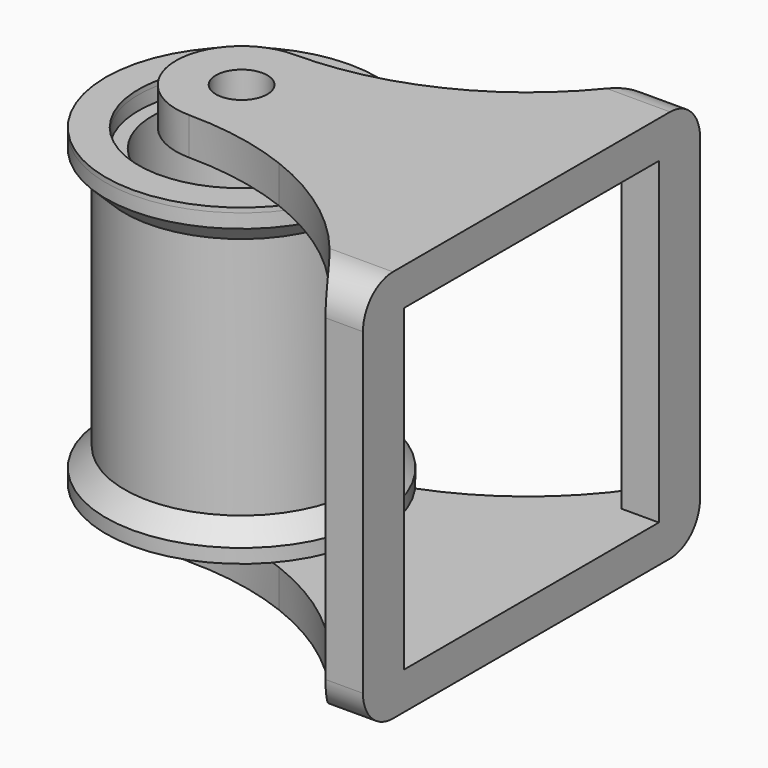
from build123d import *

# Parameters (mm, degrees)
F2_DEPTH = 0.5
F3_R     = 2.75
F4_DEPTH = 4
F6_DEPTH = 34
F7_R     = 4
F8_W     = 34
F8_H     = 34
F9_DEPTH = 4


# Not quite as in the source:
# - a feature names something its author has since deleted; it is built from what else it names


with BuildPart() as f1:
    # F0 (on Front) → F1 (revolve)
    with BuildSketch(Plane.XZ):
        Polygon((14.5, 16.5), (11, 16.5), (11, 15), (9.5, 15), (9.5, 0), (9.5, -15), (11, -15), (11, -16.5), (14.5, -16.5), (14.5, -15), (12.5, -13), (12.5, 0), (12.5, 13), (14.5, 15), align=None)
    revolve(axis=Axis((0, 0, 0.2111420035), (0, 0, -1)))


with BuildPart() as f2:
    # F2 (new): a face of the model
    f2_faces = [f1.part.faces().sort_by_distance(p)[0] for p in [
        (-14.0898780669, 0, 16.5),
    ]]
    extrude(f2_faces, amount=F2_DEPTH)


with BuildPart() as f4:
    # F3 (on face) → F4 (new body)
    with BuildSketch(Plane.XY.offset(17)):
        with BuildLine():
            ThreePointArc((11, 0), (10.1171669047, 4.3177463824), (7.6103756686, 7.9424292369))
            ThreePointArc((7.6103756686, 7.9424292369), (3.834253209, 7.2365037118), (0, 7))
            ThreePointArc((0, 7), (-4.9497474683, 4.9497474683), (-7, 0))
            ThreePointArc((-7, 0), (-4.9497474683, -4.9497474683), (0, -7))
            ThreePointArc((0, -7), (3.834253209, -7.2365037118), (7.6103756686, -7.9424292369))
            ThreePointArc((7.6103756686, -7.9424292369), (10.1171669047, -4.3177463824), (11, 0))
        make_face()
        Circle(F3_R, mode=Mode.SUBTRACT)
        with BuildLine():
            Line((26.9615242271, -22.5), (26.9615242271, 0))
            Line((26.9615242271, 0), (26.9615242271, 22.5))
            ThreePointArc((26.9615242271, 22.5), (20.2590407655, 14.4724078126), (11.2803403418, 9.1106488118))
            ThreePointArc((11.2803403418, 9.1106488118), (13.6714105885, 4.831411028), (14.5, 0))
            ThreePointArc((14.5, 0), (13.6714105885, -4.831411028), (11.2803403418, -9.1106488118))
            ThreePointArc((11.2803403418, -9.1106488118), (20.2590407655, -14.4724078126), (26.9615242271, -22.5))
        make_face()
        Polygon((26.9615242271, 22.5), (26.9615242271, 0), (26.9615242271, -22.5), (30.9615242271, -22.5), (30.9615242271, 0), (30.9615242271, 22.5), align=None)
        with BuildLine():
            ThreePointArc((14.5, 0), (13.6714105885, 4.831411028), (11.2803403418, 9.1106488118))
            ThreePointArc((11.2803403418, 9.1106488118), (9.4634017187, 8.4698546538), (7.6103756686, 7.9424292369))
            ThreePointArc((7.6103756686, 7.9424292369), (10.1171669047, 4.3177463824), (11, 0))
            ThreePointArc((11, 0), (10.1171669047, -4.3177463824), (7.6103756686, -7.9424292369))
            ThreePointArc((7.6103756686, -7.9424292369), (9.4634017187, -8.4698546538), (11.2803403418, -9.1106488118))
            ThreePointArc((11.2803403418, -9.1106488118), (13.6714105885, -4.831411028), (14.5, 0))
        make_face()
    extrude(amount=F4_DEPTH)


with BuildPart() as f5_1:
    # F5: instance of F4
    add(f4.part.mirror(Plane.XY))


with BuildPart() as f4_1:
    add(f4.part)

    add(f5_1.part)  # F6 merges F5_1
    # F3 (on face) → F6 (join, through all)
    with BuildSketch(Plane.XY.offset(17)):
        Polygon((26.9615242271, 22.5), (26.9615242271, 0), (26.9615242271, -22.5), (30.9615242271, -22.5), (30.9615242271, 0), (30.9615242271, 22.5), align=None)
    extrude(amount=-F6_DEPTH)

    # F7
    f7_edges = [f4_1.edges().sort_by_distance(p)[0] for p in [
        (28.961524, 22.5, 21),
        (28.961524, 22.5, -21),
        (28.961524, -22.5, -21),
        (28.961524, -22.5, 21),
    ]]
    fillet(f7_edges, radius=F7_R)

    # F8 (on face) → F9 (cut, through all)
    with BuildSketch(Plane.YZ.offset(30.9615242271)):
        Rectangle(F8_W, F8_H)
    extrude(amount=-F9_DEPTH, mode=Mode.SUBTRACT)


solid = Compound([f1.part, f2.part, f4_1.part])
